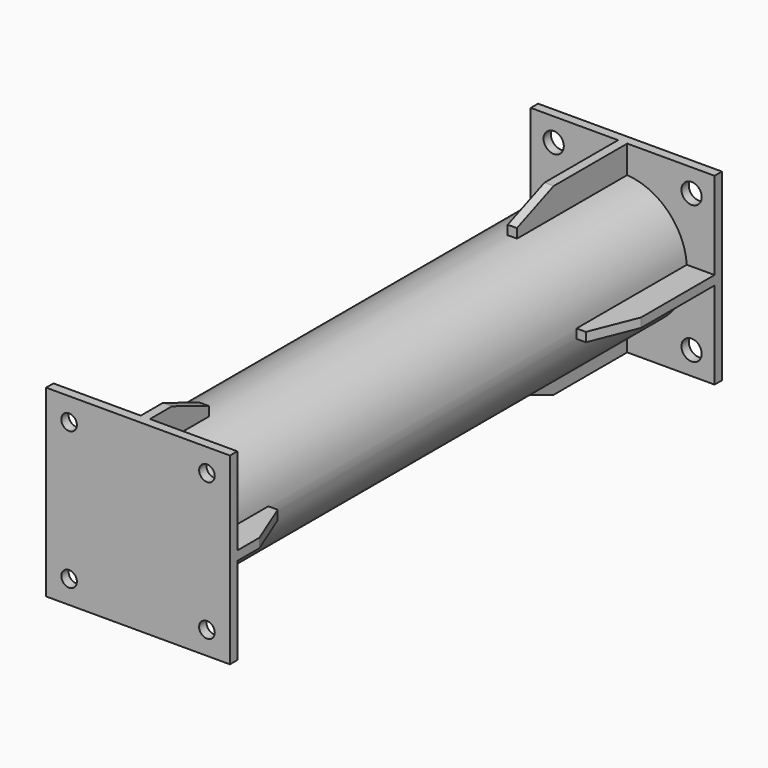
from build123d import *

# Parameters (mm, degrees)
F0_R          = 70
F0_R_2        = 65
F1_DEPTH      = 649
F2_W          = 200
F2_H          = 200
F2_R          = 11
F3_DEPTH      = 10
F4_W          = 30.1787997812
F4_H          = 10
F4_W_2        = 10
F4_H_2        = 30.1787997812
F5_DEPTH      = 150
F6_T1_DEPTH   = 269.311363913
F6_T3_DEPTH   = 269.311363913
F6_T8_DEPTH   = 269.311363913
F6_S9_R       = 70
F6_T10_DEPTH  = 139
F8_W          = 200
F8_H          = 200
F8_R          = 8.5
F9_DEPTH      = 10
F10_W         = 10
F10_H         = 30.1787997812
F10_W_2       = 30.1787997812
F10_H_2       = 10
F11_DEPTH     = 80
F12_T1_DEPTH  = 269.311363913
F12_T3_DEPTH  = 269.311363913
F12_T8_DEPTH  = 269.311363913
F12_S9_R      = 70
F12_T10_DEPTH = 139
F12_T14_DEPTH = 269.311363913
F12_S15_R     = 70
F12_T16_DEPTH = 139


# Not quite as in the source:
# - a fillet or chamfer that OpenCascade refuses, or shapes differently, is made with other operations: its cross-section is extruded or revolved along the edge and cut away or added


with BuildPart() as f1:
    # F0 (on Front) → F1 (new body)
    with BuildSketch(Plane.XZ):
        Circle(F0_R)
        Circle(F0_R_2, mode=Mode.SUBTRACT)
    extrude(amount=F1_DEPTH)

    # F2 (on Front) → F3 (join)
    with BuildSketch(Plane.XZ):
        Rectangle(F2_W, F2_H)
        with Locations((-75, -75)):
            Circle(F2_R, mode=Mode.SUBTRACT)
        with Locations((75, -75)):
            Circle(F2_R, mode=Mode.SUBTRACT)
        with Locations((-75, 75)):
            Circle(F2_R, mode=Mode.SUBTRACT)
        with Locations((75, 75)):
            Circle(F2_R, mode=Mode.SUBTRACT)
    extrude(amount=-F3_DEPTH)

    # F4 (on Front) → F5 (join)
    with BuildSketch(Plane.XZ):
        with Locations((-84.9106001094, 0)):
            Rectangle(F4_W, F4_H)
        with Locations((0, 84.9106001094)):
            Rectangle(F4_W_2, F4_H_2)
        with Locations((84.9106001094, 0)):
            Rectangle(F4_W, F4_H)
        with Locations((0, -84.9106001094)):
            Rectangle(F4_W_2, F4_H_2)
    extrude(amount=F5_DEPTH)

    # F6: chamfer of 50 x 20 on 4 edges, made by hand

    # F6_s2 → F6_t1 (cut)
    with BuildSketch(Plane.YZ.offset(-134.6556819565)):
        Polygon((-100, 100), (-150, 80), (-150, 100), align=None)
        Polygon((-100, -100), (-150, -80), (-150, -100), align=None)
    extrude(amount=F6_T1_DEPTH, mode=Mode.SUBTRACT)

    # F6_s4 → F6_t3 (cut)
    with BuildSketch(Plane.XY.offset(-134.6556819565)):
        Polygon((100, -100), (80, -150), (100, -150), align=None)
    extrude(amount=F6_T3_DEPTH, mode=Mode.SUBTRACT)


with BuildPart() as f6_tool6:
    # F6_s7 → F6_t8 (new body)
    with BuildSketch(Plane.XY.offset(134.6556819565)):
        Polygon((-100, -130), (-50, -150), (-100, -150), align=None)
    extrude(amount=-F6_T8_DEPTH)

    # F6_s9 → F6_t10 (cut, symmetric)
    with BuildSketch(Plane.XZ.offset(140)):
        Circle(F6_S9_R)
    extrude(amount=F6_T10_DEPTH, both=True, mode=Mode.SUBTRACT)


with BuildPart() as f1_1:
    add(f1.part)

    # F6_t5: cut F6_tool6
    add(f6_tool6.part, mode=Mode.SUBTRACT)

    # F8 (on offset) → F9 (join)
    with BuildSketch(Plane.XZ.offset(649)):
        Rectangle(F8_W, F8_H)
        with Locations((-75, -75)):
            Circle(F8_R, mode=Mode.SUBTRACT)
        with Locations((75, -75)):
            Circle(F8_R, mode=Mode.SUBTRACT)
        with Locations((-75, 75)):
            Circle(F8_R, mode=Mode.SUBTRACT)
        with Locations((75, 75)):
            Circle(F8_R, mode=Mode.SUBTRACT)
    extrude(amount=F9_DEPTH)

    # F10 (on face) → F11 (join)
    with BuildSketch(Plane(origin=(0, -649, 0), x_dir=(-1, 0, 0), z_dir=(0, 1, 0))):
        with Locations((0, 84.9106001094)):
            Rectangle(F10_W, F10_H)
        with Locations((84.9106001094, 0)):
            Rectangle(F10_W_2, F10_H_2)
        with Locations((0, -84.9106001094)):
            Rectangle(F10_W, F10_H)
        with Locations((-84.9106001094, 0)):
            Rectangle(F10_W_2, F10_H_2)
    extrude(amount=F11_DEPTH)

    # F12: chamfer of 20 x 50 on 4 edges, made by hand

    # F12_s2 → F12_t1 (cut)
    with BuildSketch(Plane.YZ.offset(-134.6556819565)):
        Polygon((-619, 100), (-569, 80), (-569, 100), align=None)
    extrude(amount=F12_T1_DEPTH, mode=Mode.SUBTRACT)

    # F12_s4 → F12_t3 (cut)
    with BuildSketch(Plane.XY.offset(-134.6556819565)):
        Polygon((100, -619), (80, -569), (100, -569), align=None)
    extrude(amount=F12_T3_DEPTH, mode=Mode.SUBTRACT)


with BuildPart() as f12_tool6:
    # F12_s7 → F12_t8 (new body)
    with BuildSketch(Plane.XY.offset(-134.6556819565)):
        Polygon((-100, -589), (-50, -569), (-100, -569), align=None)
    extrude(amount=F12_T8_DEPTH)

    # F12_s9 → F12_t10 (cut, symmetric)
    with BuildSketch(Plane.XZ.offset(579)):
        Circle(F12_S9_R)
    extrude(amount=F12_T10_DEPTH, both=True, mode=Mode.SUBTRACT)


with BuildPart() as f1_2:
    add(f1_1.part)

    # F12_t5: cut F12_tool6
    add(f12_tool6.part, mode=Mode.SUBTRACT)


with BuildPart() as f12_tool12:
    # F12_s13 → F12_t14 (new body)
    with BuildSketch(Plane.YZ.offset(134.6556819565)):
        Polygon((-589, -100), (-569, -50), (-569, -100), align=None)
    extrude(amount=-F12_T14_DEPTH)

    # F12_s15 → F12_t16 (cut, symmetric)
    with BuildSketch(Plane.XZ.offset(579)):
        Circle(F12_S15_R)
    extrude(amount=F12_T16_DEPTH, both=True, mode=Mode.SUBTRACT)


with BuildPart() as f1_3:
    add(f1_2.part)

    # F12_t11: cut F12_tool12
    add(f12_tool12.part, mode=Mode.SUBTRACT)


solid = f1_3.part
